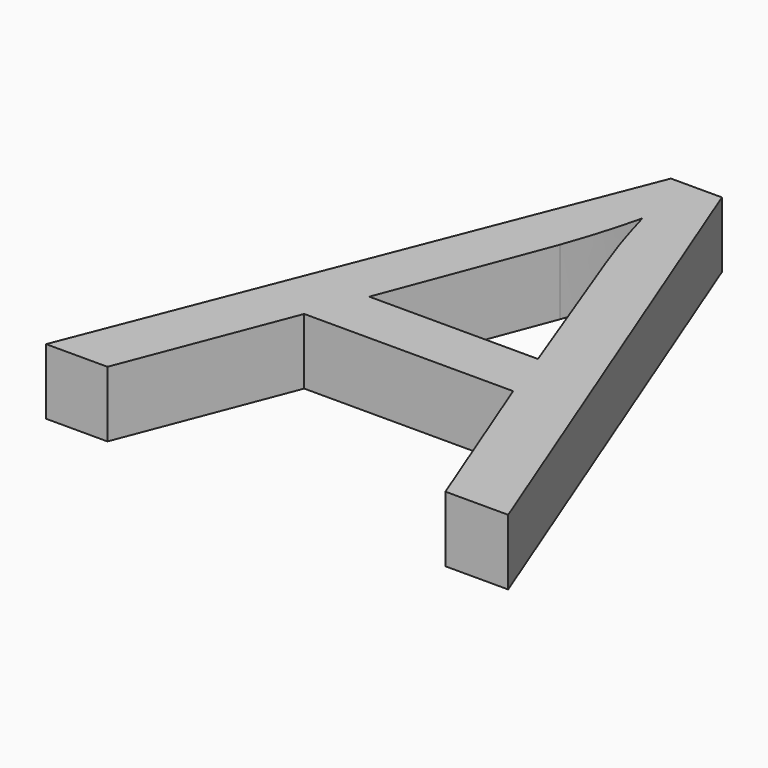
from build123d import *

# Parameters (mm, degrees)
F0_TEXT_SIZE = 282.2222222222
F1_DEPTH     = 25.4


# Not quite as in the source:
# - Text() gives the source's letters only with a copy of the font that has no kerning and outlines rounded to 1/6400 em; it was checked with that copy


with BuildPart() as f1:
    # F0 (on Top) → F1 (new body)
    with BuildSketch(Plane.XY):
        with Locations((-203.2, -13.8571532443)):
            Text('A', F0_TEXT_SIZE, font='Open Sans', text_align=(TextAlign.LEFT, TextAlign.BOTTOM))
    extrude(amount=F1_DEPTH)


solid = f1.part
